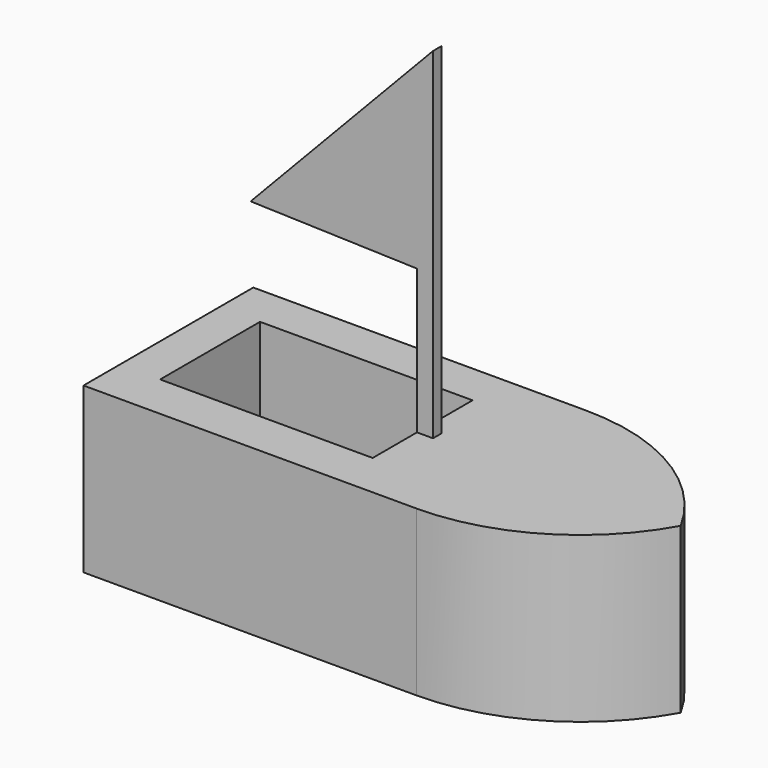
from build123d import *

# Parameters (mm, degrees)
F1_DEPTH    = 12.7
F2_T1_DEPTH = 142.3399426123
F3_DEPTH    = 0.635
F4_W        = 25.4420624115
F4_H        = 14.9451009929
F5_DEPTH    = 10.668


# Not quite as in the source:
# - a fillet or chamfer that OpenCascade refuses, or shapes differently, is made with other operations: its cross-section is extruded or revolved along the edge and cut away or added


with BuildPart() as f1:
    # F0 (on Front) → F1 (new body, symmetric)
    with BuildSketch(Plane.XZ):
        Polygon((0, 3.2491369639), (-30.2575901151, 3.2491369639), (-30.2575901151, -16.4487566799), (34.1159366071, -16.4487566799), (34.1159366071, 3.2491369639), (1.929173246, 3.2491369639), align=None)
    extrude(amount=F1_DEPTH, both=True)

    # F2: fillet of radius 24.5284097937 on 2 edges, made by hand

    # F2_s2 → F2_t1 (cut)
    with BuildSketch(Plane.XY.offset(-77.7697811642)):
        with BuildLine():
            ThreePointArc((34.1159366071, 11.8284097937), (26.9317317103, -5.5157951031), (9.5875268134, -12.7))
            Line((9.5875268134, -12.7), (34.1159366071, -12.7))
            Line((34.1159366071, -12.7), (34.1159366071, 11.8284097937))
        make_face()
        with BuildLine():
            ThreePointArc((9.5875268134, 12.7), (26.9317317103, 5.5157951031), (34.1159366071, -11.8284097937))
            Line((34.1159366071, -11.8284097937), (34.1159366071, 12.7))
            Line((34.1159366071, 12.7), (9.5875268134, 12.7))
        make_face()
    extrude(amount=F2_T1_DEPTH, mode=Mode.SUBTRACT)

    # F4 (on face) → F5 (cut)
    with BuildSketch(Plane.XY.offset(3.2491369639)):
        with Locations((-12.7083181869, 0.2053966746)):
            Rectangle(F4_W, F4_H)
    extrude(amount=-F5_DEPTH, mode=Mode.SUBTRACT)


with BuildPart() as f3:
    # F0 (on Front) → F3 (new body, symmetric)
    with BuildSketch(Plane.XZ):
        Polygon((0, 20.5101780593), (0, 3.2491369639), (1.929173246, 3.2491369639), (1.929173246, 44.0664216876), (-19.900964573, 21.119389683), align=None)
    extrude(amount=F3_DEPTH, both=True)


solid = Compound([f1.part, f3.part])
